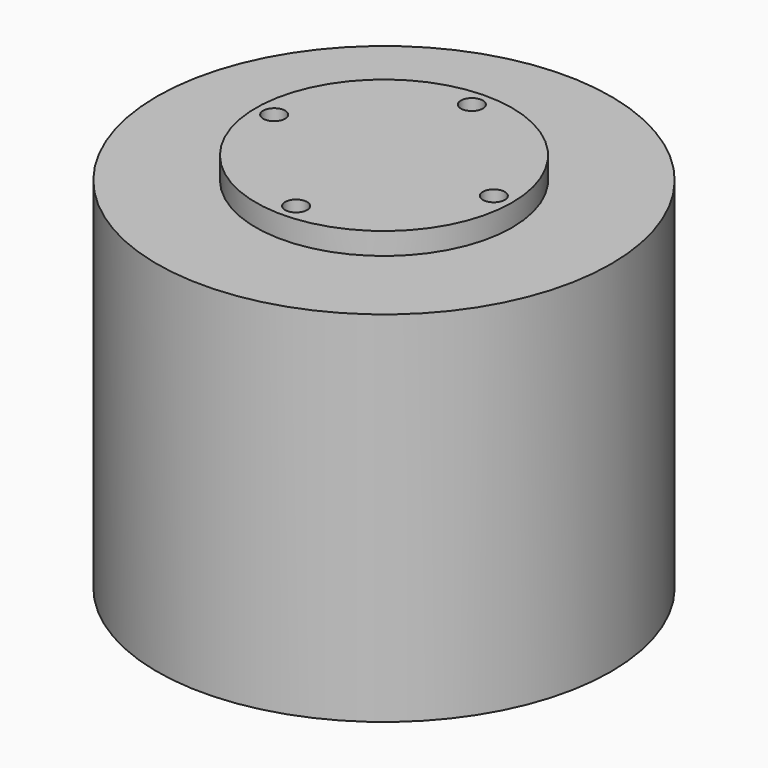
from build123d import *

# Parameters (mm, degrees)
F0_R     = 31
F1_DEPTH = 49
F2_R     = 17.5
F4_DEPTH = 52
F6_D     = 3


# Not quite as in the source:
# - the program builds the solid bodies; features that only make, move or delete a surface that nothing else refers to are left out


with BuildPart() as f1:
    # F0 (on Top) → F1 (new body)
    with BuildSketch(Plane.XY):
        Circle(F0_R)
    extrude(amount=F1_DEPTH)

    # F2 (on Top) → F4 (join)
    with BuildSketch(Plane.XY):
        Circle(F2_R)
    extrude(amount=F4_DEPTH)

    # F6 (through all)
    with Locations(Plane.XY.offset(52)):
        with Locations((0, 15), (-15, 0), (0, -15), (15, 0)):
            Hole(F6_D / 2)


solid = f1.part
